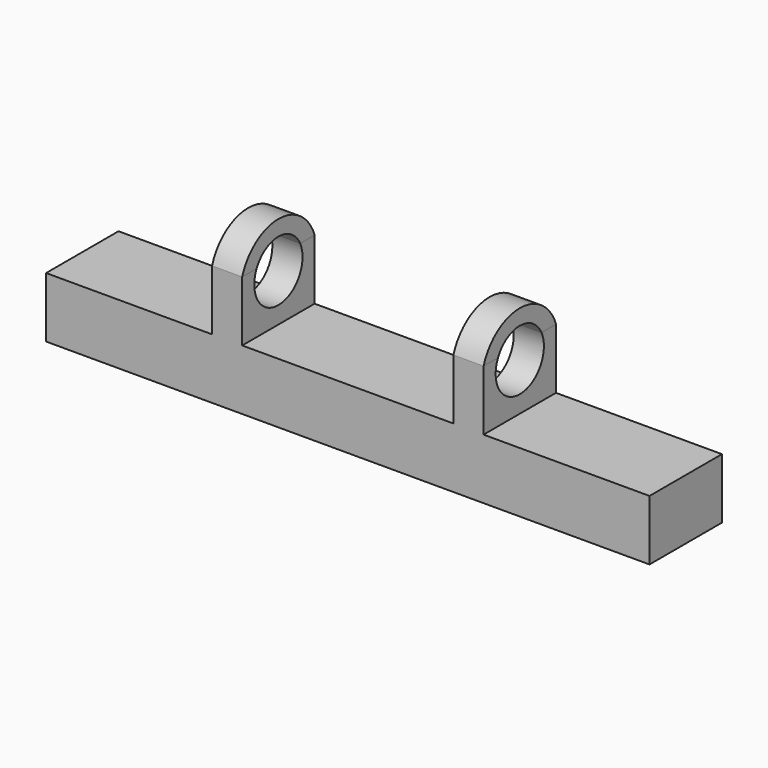
from build123d import *
from build123d import SkipClean  # not in build123d's __all__

# Parameters (mm, degrees)
F1_DEPTH = 7.62
F2_DEPTH = 7.62
F0_W     = 2.54
F0_H     = 5.08
F3_DEPTH = 7.62
F5_DEPTH = 2.54
F6_DEPTH = 36.831


# Not quite as in the source:
# - a feature names something its author has since deleted; it is built from what else it names


with BuildPart() as f1:
    # F0 (on Front) → F1 (new body)
    with BuildSketch(Plane.XZ):
        Polygon((8.89, 0), (0, 0), (-8.89, 0), (-11.43, 0), (-25.4, 0), (-25.4, -5.08), (25.4, -5.08), (25.4, 0), (11.43, 0), align=None)
    extrude(amount=F1_DEPTH)

    # F0 (on Front) → F2 (join)
    with BuildSketch(Plane.XZ):
        Polygon((8.89, 0), (0, 0), (-8.89, 0), (-11.43, 0), (-25.4, 0), (-25.4, -5.08), (25.4, -5.08), (25.4, 0), (11.43, 0), align=None)
    extrude(amount=F2_DEPTH)

    # F0 (on Front) → F3 (join)
    with BuildSketch(Plane.XZ):
        with Locations((-10.16, 2.54)):
            Rectangle(F0_W, F0_H)
        with Locations((10.16, 2.54)):
            Rectangle(F0_W, F0_H)
    extrude(amount=F3_DEPTH)

    # F4 (on face) → F5 (join)
    with BuildSketch(Plane(origin=(-11.43, 0, 0), x_dir=(0, -1, 0), z_dir=(-1, 0, 0))):
        with BuildLine():
            Line((6.1004036929, 5.08), (7.62, 5.08))
            ThreePointArc((7.62, 5.08), (3.81, 7.8260926284), (0, 5.08))
            Line((0, 5.08), (1.5195963071, 5.08))
            ThreePointArc((1.5195963071, 5.08), (3.81, 6.5219786325), (6.1004036929, 5.08))
        make_face()
    extrude(amount=-F5_DEPTH)

    # F4 (on face) → F6 (cut, through all)
    with BuildSketch(Plane(origin=(-11.43, 0, 0), x_dir=(0, -1, 0), z_dir=(-1, 0, 0))):
        with BuildLine():
            ThreePointArc((6.35, 3.9819786325), (6.2868150294, 4.5449948934), (6.1004036929, 5.08))
            Line((6.1004036929, 5.08), (1.5195963071, 5.08))
            ThreePointArc((1.5195963071, 5.08), (3.2469837391, 1.5051636031), (6.35, 3.9819786325))
        make_face()
    with SkipClean():  # cleaning this boolean's faces spoils the solid; the shape is the same uncleaned
        extrude(amount=-F6_DEPTH, mode=Mode.SUBTRACT)

    # F7: F1 across plane


with BuildPart() as f1_1:
    add(f1.part, clean=False)
    with SkipClean():  # cleaning this boolean's faces spoils the solid; the shape is the same uncleaned
        add(f1.part.mirror(Plane.YZ), clean=False)


solid = f1_1.part
